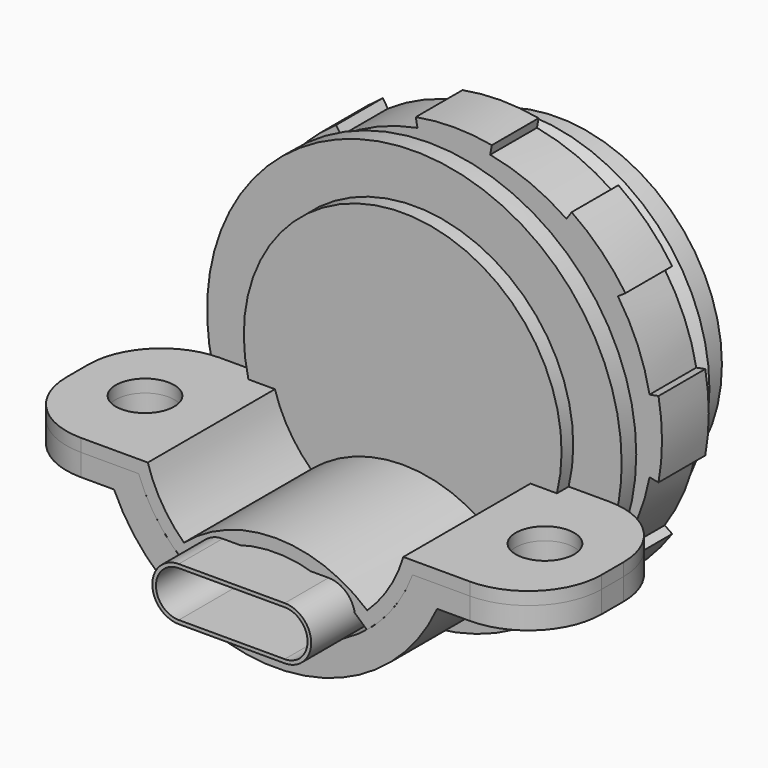
from build123d import *

# Parameters (mm, degrees)
F3_DEPTH     = 9.5
F4_T1_DEPTH  = 21.2
F4_T6_DEPTH  = 21.2
F4_S7_R      = 11.35
F4_T8_DEPTH  = 12
F4_T12_DEPTH = 21.2
F4_S13_R     = 11.35
F4_T14_DEPTH = 12
F5_R         = 1.6
F6_DEPTH     = 1.2
F8_DEPTH     = 9.5
F10_DEPTH    = 0.8
F11_R        = 4
F12_R        = 1.6
F13_DEPTH    = 0.7
F17_DEPTH    = 3.2
F19_DEPTH    = 12.5
F21_DEPTH    = 25


# Not quite as in the source:
# - a fillet or chamfer that OpenCascade refuses, or shapes differently, is made with other operations: its cross-section is extruded or revolved along the edge and cut away or added


with BuildPart() as f1:
    # F0 (on Top) → F1 (revolve)
    with BuildSketch(Plane.XY):
        Polygon((9, 9.8), (8, 9.8), (8, 0), (11.35, 0), (11.35, 1), (9, 1), (9, 2.5), (10, 3.0773502692), (9, 3.6547005384), (10, 4.2320508076), (9, 4.8094010768), (10, 5.3867513459), (9, 5.9641016151), (10, 6.5414518843), (9, 7.1188021535), (10, 7.6961524227), (9, 8.2735026919), align=None)
    revolve(axis=Axis((0, 0, 0), (0, -1, 0)))

    # F2 (on face) → F3 (join)
    with BuildSketch(Plane.XZ):
        with BuildLine():
            ThreePointArc((7.5, -2.7838821814), (0, -8), (-7.5, -2.7838821814))
            Line((-7.5, -2.7838821814), (-14.65, -2.7838821814))
            Line((-14.65, -2.7838821814), (-14.65, -3.9838821814))
            Line((-14.65, -3.9838821814), (-8.8441326745, -3.9838821814))
            ThreePointArc((-8.8441326745, -3.9838821814), (0, -9.7), (8.8441326745, -3.9838821814))
            Line((8.8441326745, -3.9838821814), (14.65, -3.9838821814))
            Line((14.65, -3.9838821814), (14.65, -2.7838821814))
            Line((14.65, -2.7838821814), (7.5, -2.7838821814))
        make_face()
    extrude(amount=F3_DEPTH)

    # F4: fillet of radius 4 on 4 edges, made by hand

    # F4_s2 → F4_t1 (cut)
    with BuildSketch(Plane.XY.offset(-13.9838821814)):
        with BuildLine():
            ThreePointArc((14.65, -5.5), (13.4784271247, -8.3284271247), (10.65, -9.5))
            Line((10.65, -9.5), (14.65, -9.5))
            Line((14.65, -9.5), (14.65, -5.5))
        make_face()
        with BuildLine():
            ThreePointArc((-14.65, -5.5), (-13.4784271247, -8.3284271247), (-10.65, -9.5))
            Line((-10.65, -9.5), (-14.65, -9.5))
            Line((-14.65, -9.5), (-14.65, -5.5))
        make_face()
    extrude(amount=F4_T1_DEPTH, mode=Mode.SUBTRACT)


with BuildPart() as f4_tool4:
    # F4_s5 → F4_t6 (new body)
    with BuildSketch(Plane.XY.offset(-13.9838821814)):
        with BuildLine():
            ThreePointArc((10.65, 0), (13.4784271247, -1.1715728753), (14.65, -4))
            Line((14.65, -4), (14.65, 0))
            Line((14.65, 0), (10.65, 0))
        make_face()
    extrude(amount=F4_T6_DEPTH)

    # F4_s7 → F4_t8 (cut, symmetric)
    with BuildSketch(Plane.XZ.offset(2)):
        Circle(F4_S7_R)
    extrude(amount=F4_T8_DEPTH, both=True, mode=Mode.SUBTRACT)


with BuildPart() as f1_1:
    add(f1.part)

    # F4_t3: cut F4_tool4
    add(f4_tool4.part, mode=Mode.SUBTRACT)


with BuildPart() as f4_tool10:
    # F4_s11 → F4_t12 (new body)
    with BuildSketch(Plane.XY.offset(7.2161178186)):
        with BuildLine():
            ThreePointArc((-10.65, 0), (-13.4784271247, -1.1715728753), (-14.65, -4))
            Line((-14.65, -4), (-14.65, 0))
            Line((-14.65, 0), (-10.65, 0))
        make_face()
    extrude(amount=-F4_T12_DEPTH)

    # F4_s13 → F4_t14 (cut, symmetric)
    with BuildSketch(Plane.XZ.offset(2)):
        Circle(F4_S13_R)
    extrude(amount=F4_T14_DEPTH, both=True, mode=Mode.SUBTRACT)


with BuildPart() as f1_2:
    add(f1_1.part)

    # F4_t9: cut F4_tool10
    add(f4_tool10.part, mode=Mode.SUBTRACT)

    # F5 (on face) → F6 (cut, through all)
    with BuildSketch(Plane.XY.offset(-2.7838821814)):
        with Locations((10.95, -4.75)):
            Circle(F5_R)
        with Locations((-10.95, -4.75)):
            Circle(F5_R)
    extrude(amount=-F6_DEPTH, mode=Mode.SUBTRACT)


with BuildPart() as f8:
    # F7 (on face) → F8 (new body)
    with BuildSketch(Plane.XZ):
        with BuildLine():
            ThreePointArc((5, -6.2449979984), (6.4851623476, -4.6843003026), (7.5, -2.7838821814))
            Line((7.5, -2.7838821814), (14.65, -2.7838821814))
            Line((14.65, -2.7838821814), (14.65, -2.0838821814))
            Line((14.65, -2.0838821814), (6.9962443535, -2.0838821814))
            ThreePointArc((6.9962443535, -2.0838821814), (6.218516923, -3.8236170412), (5.0170181209, -5.3027850394))
            ThreePointArc((5.0170181209, -5.3027850394), (0, -3.443977484), (-5.0170181209, -5.3027850394))
            ThreePointArc((-5.0170181209, -5.3027850394), (-6.218516923, -3.8236170412), (-6.9962443535, -2.0838821814))
            Line((-6.9962443535, -2.0838821814), (-14.65, -2.0838821814))
            Line((-14.65, -2.0838821814), (-14.65, -2.7838821814))
            Line((-14.65, -2.7838821814), (-7.5, -2.7838821814))
            ThreePointArc((-7.5, -2.7838821814), (-6.4851623476, -4.6843003026), (-5, -6.2449979984))
            ThreePointArc((-5, -6.2449979984), (0, -4.143977484), (5, -6.2449979984))
        make_face()
    extrude(amount=F8_DEPTH)

    # F9 (on face) → F10 (join)
    with BuildSketch(Plane(origin=(0, 0, 0), x_dir=(-1, 0, 0), z_dir=(0, 1, 0))):
        with BuildLine():
            ThreePointArc((5, -6.2449979984), (6.4851623476, -4.6843003026), (7.5, -2.7838821814))
            Line((7.5, -2.7838821814), (8.242572414, -2.7838821814))
            ThreePointArc((8.242572414, -2.7838821814), (0, 8.7), (-8.242572414, -2.7838821814))
            Line((-8.242572414, -2.7838821814), (-7.5, -2.7838821814))
            ThreePointArc((-7.5, -2.7838821814), (-6.4851623476, -4.6843003026), (-5, -6.2449979984))
            ThreePointArc((-5, -6.2449979984), (0, -4.143977484), (5, -6.2449979984))
        make_face()
    extrude(amount=-F10_DEPTH)

    # F11
    f11_edges = [f8.edges().sort_by_distance(p)[0] for p in [
        (14.65, -9.5, -2.433882),
        (14.65, 0, -2.433882),
        (-14.65, 0, -2.433882),
        (-14.65, -9.5, -2.433882),
    ]]
    fillet(f11_edges, radius=F11_R)

    # F12 (on face) → F13 (cut, through all)
    with BuildSketch(Plane.XY.offset(-2.0838821814)):
        with Locations((10.95, -4.75)):
            Circle(F12_R)
        with Locations((-10.95, -4.75)):
            Circle(F12_R)
    extrude(amount=-F13_DEPTH, mode=Mode.SUBTRACT)


with BuildPart() as f15:
    # F14 (on Top) → F15 (revolve)
    with BuildSketch(Plane.XY):
        Polygon((9.1110272543, 5.9), (10, 5.3867513459), (9, 4.8094010768), (10, 4.2320508076), (9, 3.6547005384), (10, 3.0773502692), (9.3464101615, 2.7), (11.4, 2.7), (11.4, 5.9), align=None)
    revolve(axis=Axis((0, 0, 0), (0, -1, 0)))

    # F16 (on face) → F17 (cut, through all)
    with BuildSketch(Plane(origin=(0, 5.9, 0), x_dir=(-1, 0, 0), z_dir=(0, 1, 0))):
        with BuildLine():
            Line((-1.9915654145, 10.7165137615), (-2.0829216262, 11.2080969615))
            ThreePointArc((-2.0829216262, 11.2080969615), (-4.362591129, 10.5322266706), (-6.4524733591, 9.3981693723))
            Line((-6.4524733591, 9.3981693723), (-6.1694701416, 8.9859689612))
            ThreePointArc((-6.1694701416, 8.9859689612), (-4.1712494128, 10.0702869044), (-1.9915654145, 10.7165137615))
        make_face()
        with BuildLine():
            Line((2.0829216262, 11.2080969615), (1.9915654145, 10.7165137615))
            ThreePointArc((1.9915654145, 10.7165137615), (4.1712494128, 10.0702869044), (6.1694701416, 8.9859689612))
            Line((6.1694701416, 8.9859689612), (6.4524733591, 9.3981693723))
            ThreePointArc((6.4524733591, 9.3981693723), (4.362591129, 10.5322266706), (2.0829216262, 11.2080969615))
        make_face()
        with BuildLine():
            ThreePointArc((-10.7165137615, 1.9915654145), (-10.0702869044, 4.1712494128), (-8.9859689612, 6.1694701416))
            Line((-8.9859689612, 6.1694701416), (-9.3981693723, 6.4524733591))
            ThreePointArc((-9.3981693723, 6.4524733591), (-10.5322266706, 4.362591129), (-11.2080969615, 2.0829216262))
            Line((-11.2080969615, 2.0829216262), (-10.7165137615, 1.9915654145))
        make_face()
        with BuildLine():
            ThreePointArc((-8.9859689612, -6.1694701416), (-10.0702869044, -4.1712494128), (-10.7165137615, -1.9915654145))
            Line((-10.7165137615, -1.9915654145), (-11.2080969615, -2.0829216262))
            ThreePointArc((-11.2080969615, -2.0829216262), (-10.5322266706, -4.362591129), (-9.3981693723, -6.4524733591))
            Line((-9.3981693723, -6.4524733591), (-8.9859689612, -6.1694701416))
        make_face()
        with BuildLine():
            ThreePointArc((-1.9915654145, -10.7165137615), (-4.1712494128, -10.0702869044), (-6.1694701416, -8.9859689612))
            Line((-6.1694701416, -8.9859689612), (-6.4524733591, -9.3981693723))
            ThreePointArc((-6.4524733591, -9.3981693723), (-4.362591129, -10.5322266706), (-2.0829216262, -11.2080969615))
            Line((-2.0829216262, -11.2080969615), (-1.9915654145, -10.7165137615))
        make_face()
        with BuildLine():
            ThreePointArc((6.1694701416, -8.9859689612), (4.1712494128, -10.0702869044), (1.9915654145, -10.7165137615))
            Line((1.9915654145, -10.7165137615), (2.0829216262, -11.2080969615))
            ThreePointArc((2.0829216262, -11.2080969615), (4.362591129, -10.5322266706), (6.4524733591, -9.3981693723))
            Line((6.4524733591, -9.3981693723), (6.1694701416, -8.9859689612))
        make_face()
        with BuildLine():
            ThreePointArc((10.7165137615, -1.9915654145), (10.0702869044, -4.1712494128), (8.9859689612, -6.1694701416))
            Line((8.9859689612, -6.1694701416), (9.3981693723, -6.4524733591))
            ThreePointArc((9.3981693723, -6.4524733591), (10.5322266706, -4.362591129), (11.2080969615, -2.0829216262))
            Line((11.2080969615, -2.0829216262), (10.7165137615, -1.9915654145))
        make_face()
        with BuildLine():
            ThreePointArc((8.9859689612, 6.1694701416), (10.0702869044, 4.1712494128), (10.7165137615, 1.9915654145))
            Line((10.7165137615, 1.9915654145), (11.2080969615, 2.0829216262))
            ThreePointArc((11.2080969615, 2.0829216262), (10.5322266706, 4.362591129), (9.3981693723, 6.4524733591))
            Line((9.3981693723, 6.4524733591), (8.9859689612, 6.1694701416))
        make_face()
    extrude(amount=-F17_DEPTH, mode=Mode.SUBTRACT)


with BuildPart() as f19:
    # F18 (on Front) → F19 (new body, symmetric)
    with BuildSketch(Plane.XZ):
        with BuildLine():
            Line((2.9, -4.4230315851), (-2.9, -4.4230315851))
            ThreePointArc((-2.9, -4.4230315851), (-4.35, -5.8730315851), (-2.9, -7.3230315851))
            Line((-2.9, -7.3230315851), (2.9, -7.3230315851))
            ThreePointArc((2.9, -7.3230315851), (4.35, -5.8730315851), (2.9, -4.4230315851))
        make_face()
    extrude(amount=F19_DEPTH, both=True)

    # F20 (on face) → F21 (cut, through all)
    with BuildSketch(Plane(origin=(0, 12.5, 0), x_dir=(-1, 0, 0), z_dir=(0, 1, 0))):
        with BuildLine():
            ThreePointArc((2.9, -7.1230315851), (4.15, -5.8730315851), (2.9, -4.6230315851))
            Line((2.9, -4.6230315851), (-2.9, -4.6230315851))
            ThreePointArc((-2.9, -4.6230315851), (-4.15, -5.8730315851), (-2.9, -7.1230315851))
            Line((-2.9, -7.1230315851), (2.9, -7.1230315851))
        make_face()
    extrude(amount=-F21_DEPTH, mode=Mode.SUBTRACT)


solid = Compound([f1_2.part, f8.part, f15.part, f19.part])
